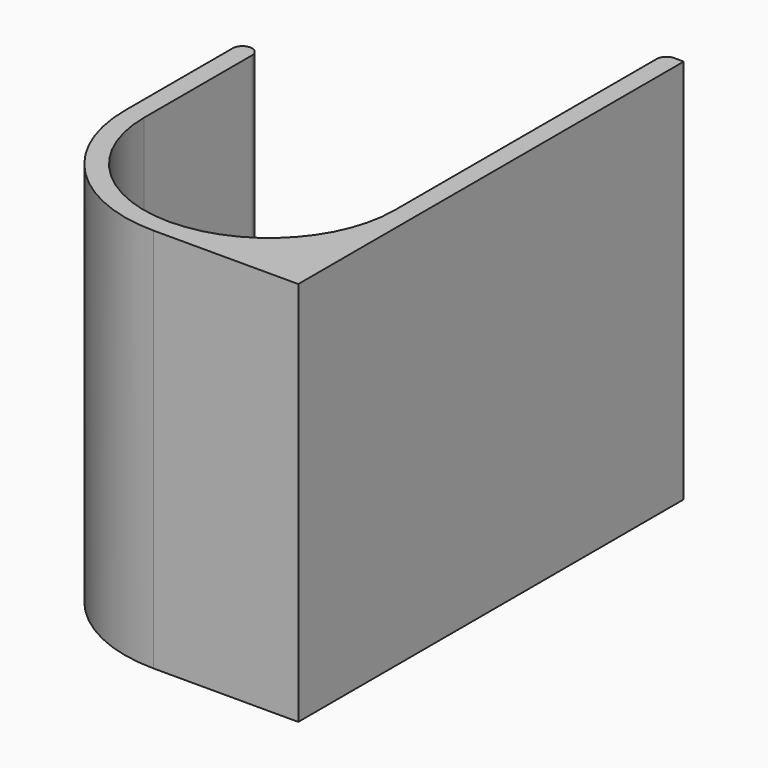
from build123d import *

# Parameters (mm, degrees)
F0_W     = 26
F0_H     = 2
F1_DEPTH = 40
F2_R     = 0.99999
F3_R     = 12.99999
F4_R     = 15


# Not quite as in the source:
# - a fillet or chamfer is up to 0.001 mm smaller than in the source, because OpenCascade refuses the exact size


with BuildPart() as f1:
    # F0 (on Top) → F1 (new body)
    with BuildSketch(Plane.XY):
        Polygon((-24.5838956386, 17.7643506003), (-26.5838956386, 17.7643506003), (-26.5838956386, -12.2356493997), (-24.5838956386, -12.2356493997), (-24.5838956386, -10.2356493997), align=None)
        with Locations((-11.5838956386, -11.2356493997)):
            Rectangle(F0_W, F0_H)
        Polygon((1.4161043614, 37.7643506003), (1.4161043614, -10.2356493997), (1.4161043614, -12.2356493997), (3.4161043614, -12.2356493997), (3.4161043614, 37.7643506003), align=None)
    extrude(amount=F1_DEPTH)

    # F2 (radius 1 in the source; OpenCascade refuses exactly that, so slightly less here)
    f2_edges = [f1.edges().sort_by_distance(p)[0] for p in [
        (-26.583896, 17.764351, 20),
        (-24.583896, 17.764351, 20),
        (1.416104, 37.764351, 20),
    ]]
    fillet(f2_edges, radius=F2_R)

    # F3 (radius 13 in the source; OpenCascade refuses exactly that, so slightly less here)
    f3_edges = [f1.edges().sort_by_distance(p)[0] for p in [
        (1.416104, -10.235649, 20),
        (-24.583896, -10.235649, 20),
    ]]
    fillet(f3_edges, radius=F3_R)

    # F4
    f4_edges = [f1.edges().sort_by_distance(p)[0] for p in [
        (-26.583896, -12.235649, 20),
    ]]
    fillet(f4_edges, radius=F4_R)


solid = f1.part
